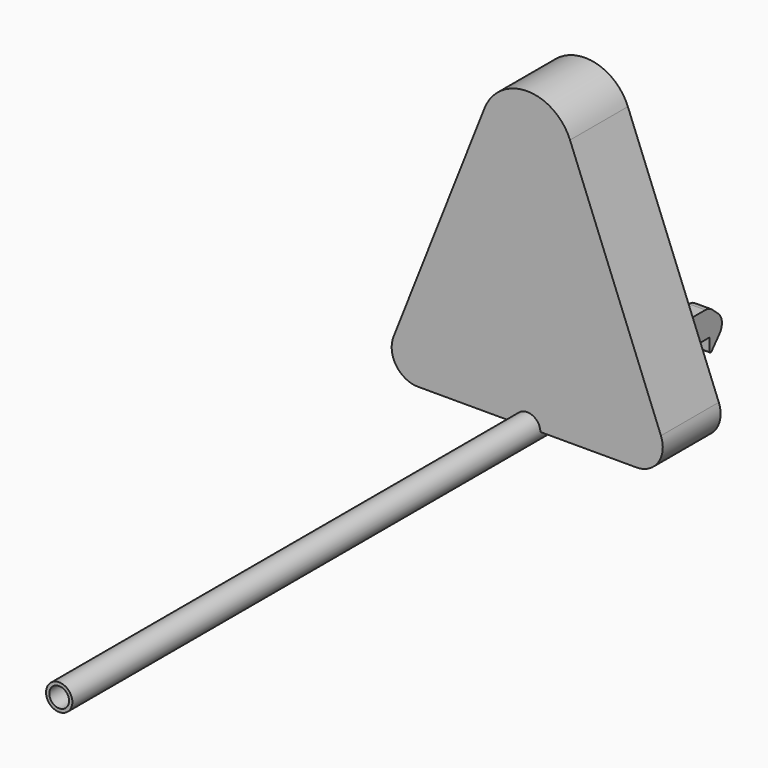
from build123d import *

# Parameters (mm, degrees)
F1_DEPTH  = 22
F2_R      = 8
F3_D      = 8
F3_DEPTH  = 15
F3_TIP    = 2.4034424761
F4_R      = 4
F4_R_2    = 3
F5_DEPTH  = 200
F7_DEPTH  = 10
F8_R      = 8
F9_R      = 2
F10_DEPTH = 28
F11_W     = 41
F11_H     = 8
F11_R     = 2
F12_DEPTH = 5
F13_R     = 3.99999
F14_R     = 0.5


# Not quite as in the source:
# - a fillet or chamfer is up to 0.001 mm smaller than in the source, because OpenCascade refuses the exact size


with BuildPart() as f1:
    # F0 (on Front) → F1 (new body)
    with BuildSketch(Plane.XZ):
        with BuildLine():
            Line((-13.0249810017, 81.1332124352), (-45, 0))
            Line((-45, 0), (45, 0))
            Line((45, 0), (13.0249810017, 81.1332124352))
            ThreePointArc((13.0249810017, 81.1332124352), (0, 90), (-13.0249810017, 81.1332124352))
        make_face()
    extrude(amount=F1_DEPTH)

    # F2
    f2_edges = [f1.edges().sort_by_distance(p)[0] for p in [
        (-45, -11, 0),
        (45, -11, 0),
    ]]
    fillet(f2_edges, radius=F2_R)

    # F3
    with Locations(Plane(origin=(0, 0, 0), x_dir=(1, 0, 0), z_dir=(0, 1, 0))):
        with Locations((0, -76)):
            Hole(F3_D / 2, depth=F3_DEPTH)
            with Locations((0, 0, -(F3_DEPTH + F3_TIP / 2))):  # 118° drill point
                Cone(0, F3_D / 2, F3_TIP, mode=Mode.SUBTRACT)


with BuildPart() as f5:
    # F4 (on Front) → F5 (new body)
    with BuildSketch(Plane.XZ):
        Circle(F4_R)
        Circle(F4_R_2, mode=Mode.SUBTRACT)
    extrude(amount=F5_DEPTH)


with BuildPart() as f7:
    # F6 (on Front) → F7 (new body)
    with BuildSketch(Plane.XZ):
        with BuildLine():
            Line((4, 31), (14, 31))
            ThreePointArc((14, 31), (0, 45), (-14, 31))
            Line((-14, 31), (-4, 31))
            ThreePointArc((-4, 31), (0, 35), (4, 31))
        make_face()
        with BuildLine():
            Line((14, 0), (14, 31))
            ThreePointArc((14, 31), (10.7470926301, 22.0278207775), (2.5, 17.225022686))
            Line((2.5, 17.225022686), (2.5, 8))
            Line((2.5, 8), (-2.5, 8))
            Line((-2.5, 8), (-2.5, 17.225022686))
            ThreePointArc((-2.5, 17.225022686), (-10.7470926301, 22.0278207775), (-14, 31))
            Line((-14, 31), (-14, 0))
            Line((-14, 0), (14, 0))
        make_face()
        with BuildLine():
            ThreePointArc((2.5, 17.225022686), (10.7470926301, 22.0278207775), (14, 31))
            Line((14, 31), (4, 31))
            ThreePointArc((4, 31), (0, 27), (-4, 31))
            Line((-4, 31), (-14, 31))
            ThreePointArc((-14, 31), (-10.7470926301, 22.0278207775), (-2.5, 17.225022686))
            Line((-2.5, 17.225022686), (-2.5, 18))
            Line((-2.5, 18), (2.5, 18))
            Line((2.5, 18), (2.5, 17.225022686))
        make_face()
    extrude(amount=F7_DEPTH)

    # F8
    f8_edges = [f7.edges().sort_by_distance(p)[0] for p in [
        (14, -5, 0),
        (-14, -5, 0),
    ]]
    fillet(f8_edges, radius=F8_R)

    # F9 (on face) → F10 (cut, through all)
    with BuildSketch(Plane.YZ.offset(14)):
        with Locations((-5, 13)):
            Circle(F9_R)
    extrude(amount=-F10_DEPTH, mode=Mode.SUBTRACT)


with BuildPart() as f12:
    # F11 (on Right) → F12 (new body)
    with BuildSketch(Plane.YZ):
        with Locations((20.5, 4)):
            Rectangle(F11_W, F11_H)
        with Locations((4, 4)):
            Circle(F11_R, mode=Mode.SUBTRACT)
        Polygon((41, 8), (41, 0), (41, -5), (47.4482121493, 2.3188773274), align=None)
    extrude(amount=F12_DEPTH)

    # F13 (radius 4 in the source; OpenCascade refuses exactly that, so slightly less here)
    f13_edges = [f12.edges().sort_by_distance(p)[0] for p in [
        (2.5, 41, 8),
        (2.5, 47.448212, 2.318877),
        (2.5, 0, 8),
        (2.5, 0, 0),
    ]]
    fillet(f13_edges, radius=F13_R)

    # F14
    f14_edges = [f12.edges().sort_by_distance(p)[0] for p in [
        (2.5, 41, -5),
    ]]
    fillet(f14_edges, radius=F14_R)


solid = Compound([f1.part, f5.part, f7.part, f12.part])
